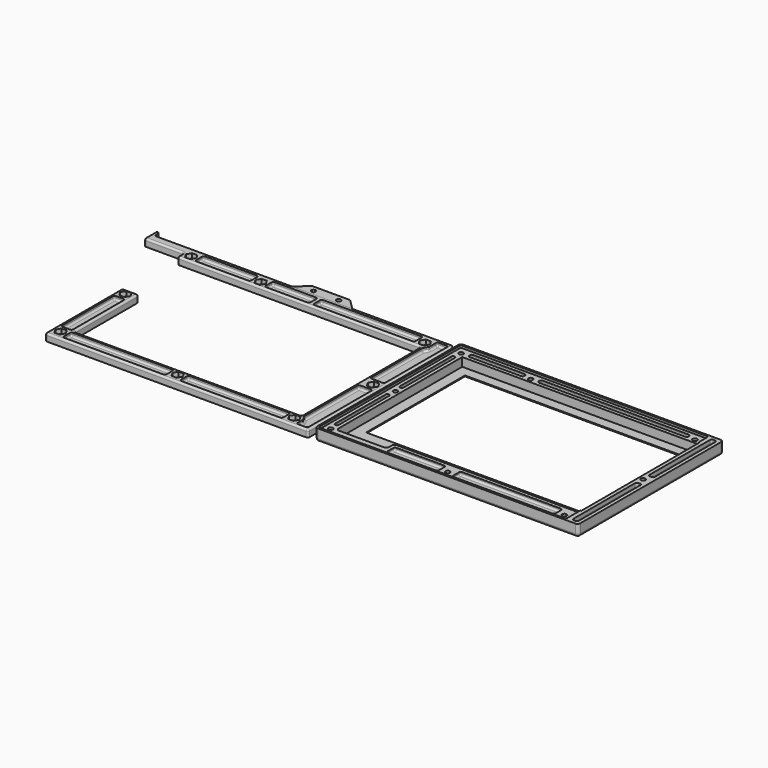
from build123d import *

# Parameters (mm, degrees)
F0_W      = 185.42
F0_H      = 128.016
F1_DEPTH  = 8.255
F2_W      = 174.625
F2_H      = 125.476
F3_DEPTH  = 1.5748
F5_DEPTH  = 7.62
F6_W      = 154.559
F6_H      = 87.122
F7_DEPTH  = 0.635
F8_R      = 1.5875
F9_DEPTH  = 8.256
F10_R     = 2.54
F11_DEPTH = 3.048
F12_R     = 1.905
F13_R     = 1.27
F14_W     = 3.81
F14_H     = 55.9308
F14_H_2   = 56.8452
F14_W_2   = 72.136
F14_H_3   = 7.493
F14_W_3   = 36.195
F14_W_4   = 105.664
F14_H_4   = 3.175
F14_W_5   = 38.862
F14_W_6   = 2.54
F14_H_5   = 47.752
F14_H_6   = 46.99
F15_DEPTH = 3.81
F16_R     = 1.26999
F17_R     = 1.5875
F18_DEPTH = 5.08
F20_DEPTH = 3.302
F21_W     = 38.862
F21_H     = 7.62
F21_W_2   = 31.623
F21_W_3   = 71.501
F21_W_4   = 72.136
F21_W_5   = 72.39
F21_W_6   = 7.62
F21_H_2   = 46.99
F22_DEPTH = 2.54
F24_DEPTH = 0.381
F25_R     = 1.26999
F26_R     = 1.524
F27_DEPTH = 5.081


# Not quite as in the source:
# - a fillet or chamfer is up to 0.001 mm smaller than in the source, because OpenCascade refuses the exact size


with BuildPart() as f1:
    # F0 (on Top) → F1 (new body)
    with BuildSketch(Plane.XY):
        with Locations((95.25, 66.548)):
            Rectangle(F0_W, F0_H)
    extrude(amount=F1_DEPTH)

    # F2 (on face) → F3 (cut)
    with BuildSketch(Plane.XY.offset(8.255)):
        with Locations((91.1225, 66.548)):
            Rectangle(F2_W, F2_H)
    extrude(amount=-F3_DEPTH, mode=Mode.SUBTRACT)

    # F4 (on face) → F5 (cut)
    with BuildSketch(Plane.XY.offset(8.255)):
        Polygon((179.07, 121.031), (11.43, 121.031), (11.43, 10.033), (46.99, 10.033), (46.99, 16.383), (179.07, 16.383), align=None)
    extrude(amount=-F5_DEPTH, mode=Mode.SUBTRACT)

    # F6 (on face) → F7 (cut, through all)
    with BuildSketch(Plane.XY.offset(0.635)):
        with Locations((96.3295, 70.358)):
            Rectangle(F6_W, F6_H)
    extrude(amount=-F7_DEPTH, mode=Mode.SUBTRACT)

    # F8 (on face) → F9 (cut, through all)
    with BuildSketch(Plane.XY.offset(8.255)):
        with Locations((8.255, 124.079)):
            Circle(F8_R)
        with Locations((57.277, 124.079)):
            Circle(F8_R)
        with Locations((173.101, 124.079)):
            Circle(F8_R)
        with Locations((173.101, 9.017)):
            Circle(F8_R)
        with Locations((8.255, 9.017)):
            Circle(F8_R)
        with Locations((8.255, 66.167)):
            Circle(F8_R)
        with Locations((90.805, 9.017)):
            Circle(F8_R)
        with Locations((182.245, 67.0052)):
            Circle(F8_R)
    extrude(amount=-F9_DEPTH, mode=Mode.SUBTRACT)

    # F10 (on face) → F11 (cut)
    with BuildSketch(Plane(origin=(0, 0, 0), x_dir=(1, 0, 0), z_dir=(0, 0, -1))):
        with Locations((173.101, -124.079)):
            Circle(F10_R)
        with Locations((182.245, -67.0052)):
            Circle(F10_R)
        with Locations((173.101, -9.017)):
            Circle(F10_R)
        with Locations((90.805, -9.017)):
            Circle(F10_R)
        with Locations((8.255, -9.017)):
            Circle(F10_R)
        with Locations((8.255, -66.167)):
            Circle(F10_R)
        with Locations((8.255, -124.079)):
            Circle(F10_R)
        with Locations((57.277, -124.079)):
            Circle(F10_R)
    extrude(amount=-F11_DEPTH, mode=Mode.SUBTRACT)

    # F12
    f12_edges = [f1.edges().sort_by_distance(p)[0] for p in [
        (187.96, 66.548, 0),
        (95.25, 2.54, 0),
        (95.25, 130.556, 0),
        (2.54, 66.548, 0),
        (2.54, 2.54, 4.1275),
        (2.54, 130.556, 4.1275),
        (187.96, 2.54, 4.1275),
        (187.96, 130.556, 4.1275),
        (11.43, 10.033, 3.6576),
        (46.99, 10.033, 3.6576),
        (46.99, 16.383, 3.6576),
    ]]
    fillet(f12_edges, radius=F12_R)

    # F13
    f13_edges = [f1.edges().sort_by_distance(p)[0] for p in [
        (3.81, 129.286, 7.4676),
        (3.81, 3.81, 7.4676),
        (178.435, 3.81, 7.4676),
        (178.435, 129.286, 7.4676),
    ]]
    fillet(f13_edges, radius=F13_R)

    # F14 (on face) → F15 (cut)
    with BuildSketch(Plane.XY.offset(8.255)):
        with Locations((183.515, 100.0506)):
            Rectangle(F14_W, F14_H)
        with Locations((183.515, 33.5026)):
            Rectangle(F14_W, F14_H_2)
        with Locations((131.953, 10.0965)):
            Rectangle(F14_W_2, F14_H_3)
        with Locations((67.6275, 10.0965)):
            Rectangle(F14_W_3, F14_H_3)
        with Locations((115.189, 125.1585)):
            Rectangle(F14_W_4, F14_H_4)
        with Locations((32.766, 125.1585)):
            Rectangle(F14_W_5, F14_H_4)
        with Locations((7.62, 95.123)):
            Rectangle(F14_W_6, F14_H_5)
        with Locations((7.62, 37.592)):
            Rectangle(F14_W_6, F14_H_6)
    extrude(amount=-F15_DEPTH, mode=Mode.SUBTRACT)

    # F16 (radius 1.27 in the source; OpenCascade refuses exactly that, so slightly less here)
    f16_edges = [f1.edges().sort_by_distance(p)[0] for p in [
        (185.42, 61.9252, 6.35),
        (181.61, 61.9252, 6.35),
        (181.61, 33.5026, 4.445),
        (183.515, 61.9252, 4.445),
        (185.42, 33.5026, 4.445),
        (185.42, 5.08, 6.35),
        (183.515, 5.08, 4.445),
        (181.61, 5.08, 6.35),
        (181.61, 72.0852, 6.35),
        (181.61, 100.0506, 4.445),
        (185.42, 100.0506, 4.445),
        (185.42, 72.0852, 6.35),
        (183.515, 72.0852, 4.445),
        (185.42, 128.016, 6.35),
        (183.515, 128.016, 4.445),
        (181.61, 128.016, 6.35),
        (168.021, 126.746, 5.5626),
        (168.021, 125.1585, 4.445),
        (115.189, 126.746, 4.445),
        (168.021, 123.571, 5.5626),
        (62.357, 125.1585, 4.445),
        (62.357, 126.746, 5.5626),
        (62.357, 123.571, 5.5626),
        (13.335, 123.571, 5.5626),
        (13.335, 125.1585, 4.445),
        (32.766, 123.571, 4.445),
        (13.335, 126.746, 5.5626),
        (52.197, 125.1585, 4.445),
        (52.197, 126.746, 5.5626),
        (32.766, 126.746, 4.445),
        (52.197, 123.571, 5.5626),
        (6.35, 118.999, 5.5626),
        (7.62, 118.999, 4.445),
        (8.89, 118.999, 5.5626),
        (8.89, 95.123, 4.445),
        (8.89, 61.087, 5.5626),
        (8.89, 37.592, 4.445),
        (7.62, 61.087, 4.445),
        (6.35, 61.087, 5.5626),
        (6.35, 95.123, 4.445),
        (6.35, 71.247, 5.5626),
        (7.62, 71.247, 4.445),
        (8.89, 71.247, 5.5626),
        (8.89, 14.097, 5.5626),
        (7.62, 14.097, 4.445),
        (6.35, 14.097, 5.5626),
        (6.35, 37.592, 4.445),
        (49.53, 6.35, 5.5626),
        (49.53, 10.0965, 4.445),
        (67.6275, 6.35, 4.445),
        (49.53, 13.843, 5.5626),
        (67.6275, 13.843, 4.445),
        (131.953, 13.843, 4.445),
        (95.885, 10.0965, 4.445),
        (131.953, 6.35, 4.445),
        (168.021, 10.0965, 4.445),
        (95.885, 6.35, 5.5626),
        (85.725, 10.0965, 4.445),
        (85.725, 6.35, 5.5626),
        (85.725, 13.843, 5.5626),
        (95.885, 13.843, 5.5626),
        (168.021, 6.35, 5.5626),
        (168.021, 13.843, 5.5626),
    ]]
    fillet(f16_edges, radius=F16_R)


with BuildPart() as f18:
    # F17 (on Top) → F18 (new body)
    with BuildSketch(Plane.XY):
        Polygon((-187.96, 70.612), (-187.96, 2.54), (-2.54, 2.54), (-2.54, 130.556), (-73.66, 130.556), (-116.84, 130.556), (-187.96, 130.556), (-213.36, 130.556), (-213.36, 135.001), (-215.9, 135.001), (-215.9, 124.841), (-187.96, 124.841), (-187.96, 119.126), (-16.256, 119.126), (-16.256, 13.97), (-176.53, 13.97), (-176.53, 70.612), align=None)
        with Locations((-182.245, 9.017)):
            Circle(F17_R, mode=Mode.SUBTRACT)
        with Locations((-182.245, 66.167)):
            Circle(F17_R, mode=Mode.SUBTRACT)
        with Locations((-99.695, 9.017)):
            Circle(F17_R, mode=Mode.SUBTRACT)
        with Locations((-17.399, 9.017)):
            Circle(F17_R, mode=Mode.SUBTRACT)
        with Locations((-8.255, 67.0052)):
            Circle(F17_R, mode=Mode.SUBTRACT)
        with Locations((-182.245, 124.079)):
            Circle(F17_R, mode=Mode.SUBTRACT)
        with Locations((-133.223, 124.079)):
            Circle(F17_R, mode=Mode.SUBTRACT)
        with Locations((-17.399, 124.079)):
            Circle(F17_R, mode=Mode.SUBTRACT)
        Polygon((-116.84, 130.556), (-73.66, 130.556), (-82.55, 139.446), (-107.95, 139.446), align=None)
    extrude(amount=F18_DEPTH)

    # F19 (on face) → F20 (cut)
    with BuildSketch(Plane.XY.offset(5.08)):
        Polygon((-180.4119128953, 120.904), (-178.5788257906, 124.079), (-180.4119128953, 127.254), (-184.0780871047, 127.254), (-185.9111742094, 124.079), (-184.0780871047, 120.904), align=None)
        Polygon((-131.3899128953, 120.904), (-129.5568257906, 124.079), (-131.3899128953, 127.254), (-135.0560871047, 127.254), (-136.8891742094, 124.079), (-135.0560871047, 120.904), align=None)
        Polygon((-15.5659128953, 120.904), (-13.7328257906, 124.079), (-15.5659128953, 127.254), (-19.2320871047, 127.254), (-21.0651742094, 124.079), (-19.2320871047, 120.904), align=None)
        Polygon((-6.4219128953, 63.8302), (-4.5888257906, 67.0052), (-6.4219128953, 70.1802), (-10.0880871047, 70.1802), (-11.9211742094, 67.0052), (-10.0880871047, 63.8302), align=None)
        Polygon((-15.5659128953, 5.842), (-13.7328257906, 9.017), (-15.5659128953, 12.192), (-19.2320871047, 12.192), (-21.0651742094, 9.017), (-19.2320871047, 5.842), align=None)
        Polygon((-97.8619128953, 5.842), (-96.0288257906, 9.017), (-97.8619128953, 12.192), (-101.5280871047, 12.192), (-103.3611742094, 9.017), (-101.5280871047, 5.842), align=None)
        Polygon((-180.4119128953, 5.842), (-178.5788257906, 9.017), (-180.4119128953, 12.192), (-184.0780871047, 12.192), (-185.9111742094, 9.017), (-184.0780871047, 5.842), align=None)
        Polygon((-180.4119128953, 62.992), (-178.5788257906, 66.167), (-180.4119128953, 69.342), (-184.0780871047, 69.342), (-185.9111742094, 66.167), (-184.0780871047, 62.992), align=None)
    extrude(amount=-F20_DEPTH, mode=Mode.SUBTRACT)

    # F21 (on face) → F22 (cut)
    with BuildSketch(Plane.XY.offset(5.08)):
        with Locations((-157.734, 124.841)):
            Rectangle(F21_W, F21_H)
        with Locations((-112.3315, 124.841)):
            Rectangle(F21_W_2, F21_H)
        with Locations((-58.2295, 124.841)):
            Rectangle(F21_W_3, F21_H)
        Polygon((-4.445, 128.651), (-12.319, 128.651), (-12.319, 121.4478181024), (-14.351, 117.9282908615), (-14.351, 72.0852), (-4.445, 72.0852), align=None)
        Polygon((-4.445, 4.445), (-4.445, 61.9252), (-14.351, 61.9252), (-14.351, 13.97), (-12.319, 10.450472759), (-12.319, 4.445), align=None)
        with Locations((-58.547, 8.255)):
            Rectangle(F21_W_4, F21_H)
        with Locations((-140.97, 8.255)):
            Rectangle(F21_W_5, F21_H)
        with Locations((-182.245, 37.592)):
            Rectangle(F21_W_6, F21_H_2)
    extrude(amount=-F22_DEPTH, mode=Mode.SUBTRACT)

    # F23 (on face) → F24 (cut)
    with BuildSketch(Plane.XY.offset(5.08)):
        Polygon((-82.55, 139.446), (-107.95, 139.446), (-116.84, 130.556), (-73.66, 130.556), align=None)
    extrude(amount=-F24_DEPTH, mode=Mode.SUBTRACT)

    # F25 (radius 1.27 in the source; OpenCascade refuses exactly that, so slightly less here)
    f25_edges = [f18.edges().sort_by_distance(p)[0] for p in [
        (-138.303, 121.031, 3.81),
        (-138.303, 128.651, 3.81),
        (-22.479, 128.651, 3.81),
        (-177.165, 128.651, 3.81),
        (-128.143, 121.031, 3.81),
        (-177.165, 121.031, 3.81),
        (-4.445, 72.0852, 3.81),
        (-4.445, 4.445, 3.81),
        (-12.319, 10.450473, 3.81),
        (-14.351, 72.0852, 3.81),
        (-14.351, 13.97, 3.81),
        (-12.319, 4.445, 3.81),
        (-4.445, 61.9252, 3.81),
        (-4.445, 128.651, 3.81),
        (-12.319, 121.447818, 3.81),
        (-14.351, 117.928291, 3.81),
        (-12.319, 128.651, 3.81),
        (-14.351, 61.9252, 3.81),
        (-94.615, 4.445, 3.81),
        (-177.165, 4.445, 3.81),
        (-94.615, 12.065, 3.81),
        (-177.165, 12.065, 3.81),
        (-22.479, 12.065, 3.81),
        (-104.775, 12.065, 3.81),
        (-22.479, 4.445, 3.81),
        (-104.775, 4.445, 3.81),
        (-178.435, 14.097, 3.81),
        (-186.055, 14.097, 3.81),
        (-178.435, 61.087, 3.81),
        (-186.055, 61.087, 3.81),
        (-178.435, 37.592, 2.54),
        (-182.245, 61.087, 2.54),
        (-186.055, 37.592, 2.54),
        (-182.245, 14.097, 2.54),
        (-140.97, 12.065, 2.54),
        (-177.165, 8.255, 2.54),
        (-140.97, 4.445, 2.54),
        (-104.775, 8.255, 2.54),
        (-58.547, 12.065, 2.54),
        (-94.615, 8.255, 2.54),
        (-58.547, 4.445, 2.54),
        (-22.479, 8.255, 2.54),
        (-4.445, 33.1851, 2.54),
        (-9.398, 61.9252, 2.54),
        (-14.351, 37.9476, 2.54),
        (-13.335, 12.210236, 2.54),
        (-12.319, 7.447736, 2.54),
        (-8.382, 4.445, 2.54),
        (-8.382, 128.651, 2.54),
        (-12.319, 125.049409, 2.54),
        (-13.335, 119.688054, 2.54),
        (-14.351, 95.006745, 2.54),
        (-9.398, 72.0852, 2.54),
        (-4.445, 100.3681, 2.54),
        (-22.479, 124.841, 2.54),
        (-58.2295, 128.651, 2.54),
        (-93.98, 124.841, 2.54),
        (-58.2295, 121.031, 2.54),
        (-157.734, 128.651, 2.54),
        (-177.165, 124.841, 2.54),
        (-157.734, 121.031, 2.54),
        (-138.303, 124.841, 2.54),
        (-187.96, 2.54, 2.54),
        (-187.96, 70.612, 2.54),
        (-176.53, 70.612, 2.54),
        (-176.53, 13.97, 2.54),
        (-16.256, 13.97, 2.54),
        (-16.256, 119.126, 2.54),
        (-187.96, 119.126, 2.54),
        (-116.84, 130.556, 2.3495),
        (-73.66, 130.556, 2.3495),
        (-2.54, 130.556, 2.54),
        (-96.52, 128.651, 3.81),
        (-93.98, 121.031, 3.81),
        (-95.25, 139.446, 4.699),
        (-187.96, 36.576, 5.08),
        (-95.25, 2.54, 5.08),
        (-182.245, 70.612, 5.08),
        (-176.53, 42.291, 5.08),
        (-187.96, 121.9835, 5.08),
        (-2.54, 66.548, 5.08),
        (-2.54, 2.54, 2.54),
        (-215.9, 129.921, 5.08),
        (-213.36, 130.556, 2.54),
        (-213.36, 135.001, 2.54),
        (-215.9, 135.001, 2.54),
        (-215.9, 124.841, 2.54),
        (-96.393, 13.97, 5.08),
        (-16.256, 66.548, 5.08),
        (-102.108, 119.126, 5.08),
        (-187.96, 124.841, 2.54),
        (-201.93, 124.841, 5.08),
        (-93.98, 128.651, 3.81),
        (-22.479, 121.031, 3.81),
        (-128.143, 128.651, 3.81),
        (-128.143, 124.841, 2.54),
        (-112.3315, 128.651, 2.54),
        (-112.3315, 121.031, 2.54),
        (-96.52, 124.841, 2.54),
        (-96.52, 121.031, 3.81),
    ]]
    fillet(f25_edges, radius=F25_R)

    # F26 (on face) → F27 (cut, through all)
    with BuildSketch(Plane.XY.offset(5.08)):
        with Locations((-104.14, 134.366)):
            Circle(F26_R)
        with Locations((-86.36, 134.366)):
            Circle(F26_R)
    extrude(amount=-F27_DEPTH, mode=Mode.SUBTRACT)


solid = Compound([f1.part, f18.part])
